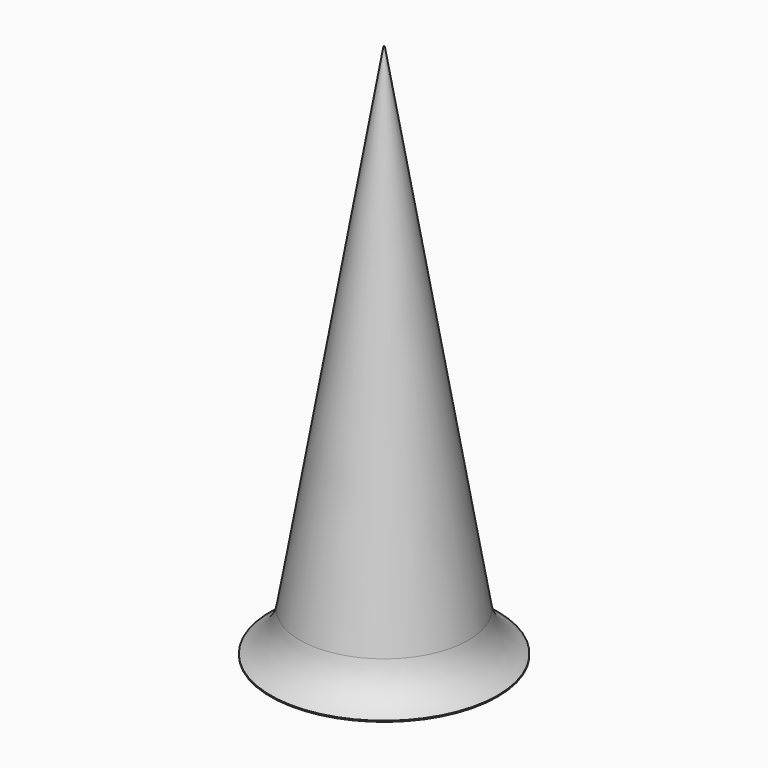
from build123d import *

# Parameters (mm, degrees)
F0_R     = 85
F2_R     = 0.5
F4_R     = 105.9677495378
F5_DEPTH = 1


# Not quite as in the source:
# - a fillet or chamfer that OpenCascade refuses, or shapes differently, is made with other operations: its cross-section is extruded or revolved along the edge and cut away or added


with BuildPart() as f3:
    # F0 (on Top) → F3 section 0
    with BuildSketch(Plane.XY):
        Circle(F0_R)
    # F2 (on offset) → F3 section 1
    with BuildSketch(Plane.XY.offset(500)):
        Circle(F2_R)
    loft()

    # F4 (on Top) → F5 (join)
    with BuildSketch(Plane.XY):
        Circle(F4_R)
    extrude(amount=F5_DEPTH)

    # F6: fillet of radius 50 on 1 edges, made by hand

    # F6_s1 → F6_t2 (revolve)
    with BuildSketch(Plane.XZ):
        with BuildLine():
            ThreePointArc((105.9677495378, 1), (87.890537333, 15.9884437146), (78.6495736084, 37.5764875242))
            Line((78.6495736084, 37.5764875242), (84.831, 1))
            Line((84.831, 1), (105.9677495378, 1))
        make_face()
    revolve(axis=Axis((0, 0, 1), (0, 0, 1)))


solid = f3.part
